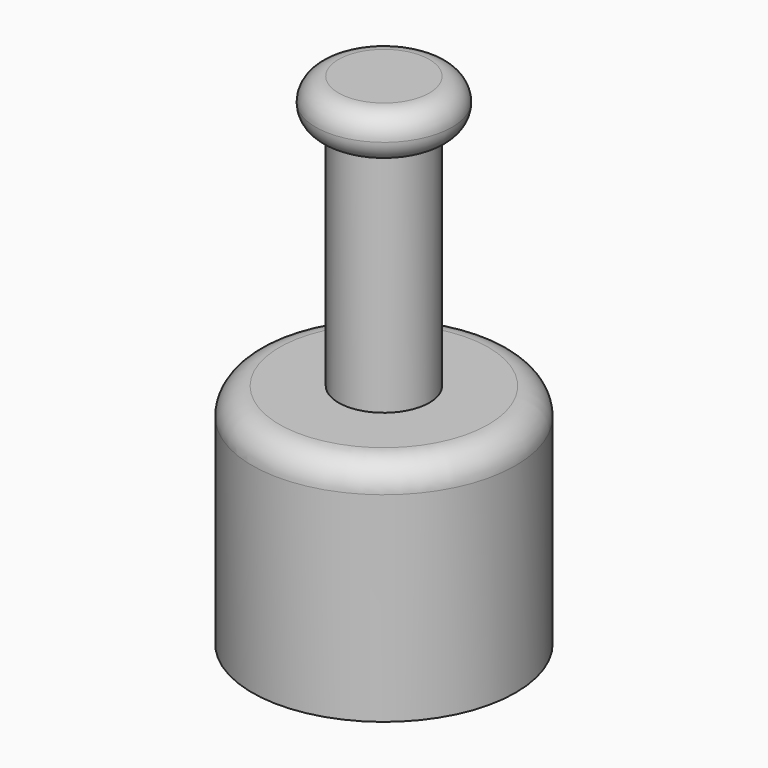
from build123d import *

# Parameters (mm, degrees)
F0_R     = 14.5
F1_DEPTH = 25
F2_R     = 5
F3_DEPTH = 25
F4_R     = 7.5
F5_DEPTH = 5
F6_R     = 2.49999
F7_R     = 3
F8_R     = 11.75
F9_DEPTH = 22.5


# Not quite as in the source:
# - a fillet or chamfer is up to 0.001 mm smaller than in the source, because OpenCascade refuses the exact size


with BuildPart() as f1:
    # F0 (on Top) → F1 (new body)
    with BuildSketch(Plane.XY):
        Circle(F0_R)
    extrude(amount=F1_DEPTH)

    # F2 (on face) → F3 (join)
    with BuildSketch(Plane.XY.offset(25)):
        Circle(F2_R)
    extrude(amount=F3_DEPTH)

    # F4 (on face) → F5 (join)
    with BuildSketch(Plane.XY.offset(50)):
        Circle(F4_R)
    extrude(amount=F5_DEPTH)

    # F6 (radius 2.5 in the source; OpenCascade refuses exactly that, so slightly less here)
    f6_edges = [f1.edges().sort_by_distance(p)[0] for p in [
        (-7.5, 0, 50),
        (-7.5, 0, 55),
    ]]
    fillet(f6_edges, radius=F6_R)

    # F7
    f7_edges = [f1.edges().sort_by_distance(p)[0] for p in [
        (-14.5, 0, 25),
    ]]
    fillet(f7_edges, radius=F7_R)

    # F8 (on face) → F9 (cut)
    with BuildSketch(Plane(origin=(0, 0, 0), x_dir=(1, 0, 0), z_dir=(0, 0, -1))):
        Circle(F8_R)
    extrude(amount=-F9_DEPTH, mode=Mode.SUBTRACT)


solid = f1.part
